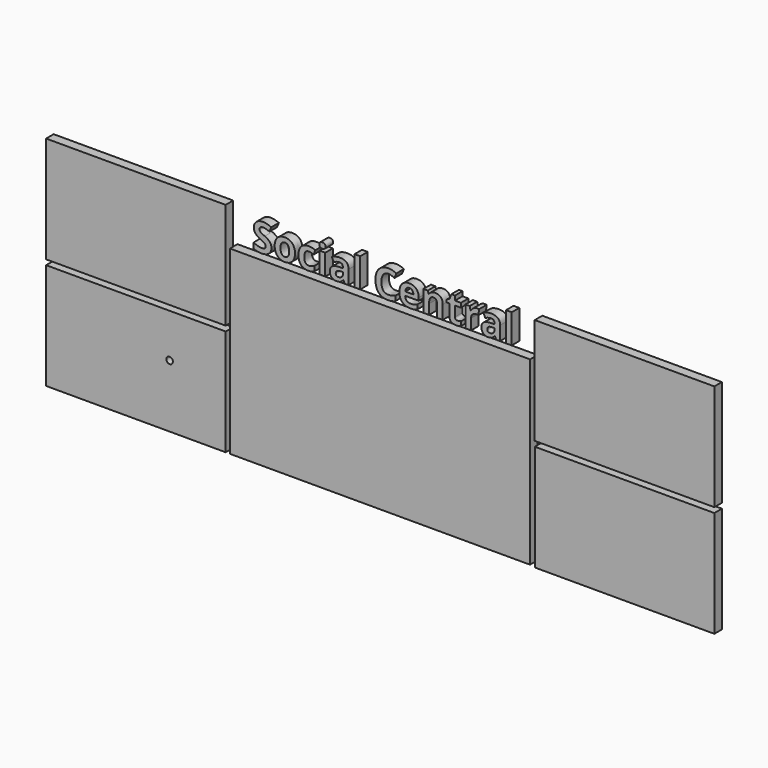
from build123d import *

# Parameters (mm, degrees)
F0_W         = 965.2
F0_H         = 571.5
F0_W_2       = 732.6093316078
F0_H_2       = 186.2565875053
F0_W_3       = 1612.9
F0_H_3       = 971.55
F0_R         = 17.5605434377
F1_TEXT_SIZE = 206.5708608659
F2_DEPTH     = 50.8


# Not quite as in the source:
# - Text() gives the source's letters only with a copy of the font that has no kerning and outlines rounded to 1/6400 em; it was checked with that copy


with BuildPart() as f2:
    # F0 (on Front) + F1 (on Front) → F2 (new body)
    with BuildSketch(Plane.XZ):
        with Locations((-1329.3491904736, 422.8918640971)):
            Rectangle(F0_W, F0_H)
        with Locations((-1329.093783617, -176.2151806712)):
            Rectangle(F0_W, F0_H)
        with Locations((-1322.9493796825, -173.4224706888)):
            Rectangle(F0_W_2, F0_H_2, mode=Mode.SUBTRACT)
        with Locations((-17.3666588962, 23.8098193288)):
            Rectangle(F0_W_3, F0_H_3)
        with Locations((-1322.9493796825, -173.4224706888)):
            Rectangle(F0_W_2, F0_H_2)
        with Locations((-1147.8682756424, -125.4151806712)):
            Circle(F0_R, mode=Mode.SUBTRACT)
        with Locations((1296.8802181105, 418.0487339256)):
            Rectangle(F0_W, F0_H)
        with Locations((1297.135624967, -181.0583108427)):
            Rectangle(F0_W, F0_H)
    with BuildSketch(Plane.XZ):
        with Locations((-706.3931010466, 543.5973672807)):
            Text('Social Central', F1_TEXT_SIZE, font='Open Sans', font_style=FontStyle.BOLD, text_align=(TextAlign.LEFT, TextAlign.BOTTOM))
    extrude(amount=F2_DEPTH)


solid = f2.part
